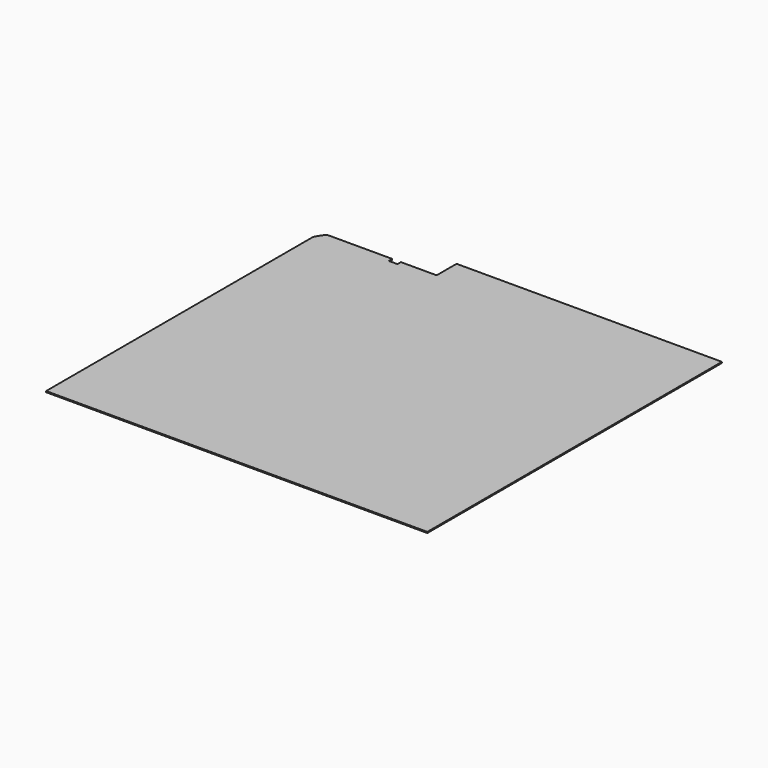
from build123d import *

# Parameters (mm, degrees)
F0_R     = 685.2304837253
F2_DEPTH = 25.4


# Not quite as in the source:
# - the program builds the solid bodies; features that only make, move or delete a surface that nothing else refers to are left out


with BuildPart() as f2:
    # F0 (on Top) → F2 (new body)
    with BuildSketch(Plane.XY):
        with BuildLine():
            Line((4934.2064314485, -2623.8248911343), (4934.2064314485, 6012.1751088657))
            Line((4934.2064314485, 6012.1751088657), (-1288.7935685515, 6012.1751088657))
            Line((-1288.7935685515, 6012.1751088657), (-1288.7935685515, 5427.9751088657))
            Line((-1288.7935685515, 5427.9751088657), (-2126.9935685515, 5427.9751088657))
            Line((-2126.9935685515, 5427.9751088657), (-2126.9935685515, 5326.3751088657))
            Line((-2126.9935685515, 5326.3751088657), (-2330.1935685515, 5326.3751088657))
            Line((-2330.1935685515, 5326.3751088657), (-2330.1935685515, 5427.9751088657))
            Line((-2330.1935685515, 5427.9751088657), (-2832.8617031592, 5427.9751088657))
            ThreePointArc((-2832.8617031592, 5427.9751088657), (-2679.6080274317, 5196.4381140006), (-2625.8343083567, 4924.033164978))
            ThreePointArc((-2625.8343083567, 4924.033164978), (-3204.9226388633, 4220.5397003228), (-4006.5935685515, 4653.6333043329))
            Line((-4006.5935685515, 4653.6333043329), (-4006.5935685515, -2623.8248911343))
            Line((-4006.5935685515, -2623.8248911343), (547.2349236927, -2623.8248911343))
            ThreePointArc((547.2349236927, -2623.8248911343), (993.2484493325, -1608.5916420747), (1868.1852008655, -2289.8495197296))
            ThreePointArc((1868.1852008655, -2289.8495197296), (1846.7485049438, -2462.0916976859), (1783.7463308849, -2623.8248911343))
            Line((1783.7463308849, -2623.8248911343), (2002.3317513014, -2623.8248911343))
            ThreePointArc((2002.3317513014, -2623.8248911343), (2539.4671679111, -1645.2150017176), (3399.7739963066, -2356.5967082977))
            ThreePointArc((3399.7739963066, -2356.5967082977), (3386.8840068426, -2492.631840649), (3348.6728492235, -2623.8248911343))
            Line((3348.6728492235, -2623.8248911343), (4934.2064314486, -2623.8248911343))
        make_face()
        with Locations((4180.0508499146, 5218.0252075195)):
            Circle(F0_R, mode=Mode.SUBTRACT)
        with BuildLine():
            ThreePointArc((-2625.8343083567, 4924.033164978), (-2679.6080274317, 5196.4381140006), (-2832.8617031592, 5427.9751088657))
            Line((-2832.8617031592, 5427.9751088657), (-3852.5197093468, 5427.9751088657))
            ThreePointArc((-3852.5197093468, 5427.9751088657), (-3941.061075774, 5318.7938470176), (-4006.5935685515, 5194.4330256231))
            Line((-4006.5935685515, 5194.4330256231), (-4006.5935685515, 4653.6333043329))
            ThreePointArc((-4006.5935685515, 4653.6333043329), (-3204.9226388633, 4220.5397003228), (-2625.8343083567, 4924.033164978))
        make_face()
        with Locations((4180.0508499146, 5218.0252075195)):
            Circle(F0_R)
        with BuildLine():
            Line((2002.3317513014, -2623.8248911343), (3348.6728492235, -2623.8248911343))
            ThreePointArc((3348.6728492235, -2623.8248911343), (3386.8840068426, -2492.631840649), (3399.7739963066, -2356.5967082977))
            ThreePointArc((3399.7739963066, -2356.5967082977), (2539.4671679111, -1645.2150017176), (2002.3317513014, -2623.8248911343))
        make_face()
        with BuildLine():
            Line((547.2349236927, -2623.8248911343), (1783.7463308849, -2623.8248911343))
            ThreePointArc((1783.7463308849, -2623.8248911343), (1846.7485049438, -2462.0916976859), (1868.1852008655, -2289.8495197296))
            ThreePointArc((1868.1852008655, -2289.8495197296), (993.2484493325, -1608.5916420747), (547.2349236927, -2623.8248911343))
        make_face()
    extrude(amount=F2_DEPTH)


solid = f2.part
